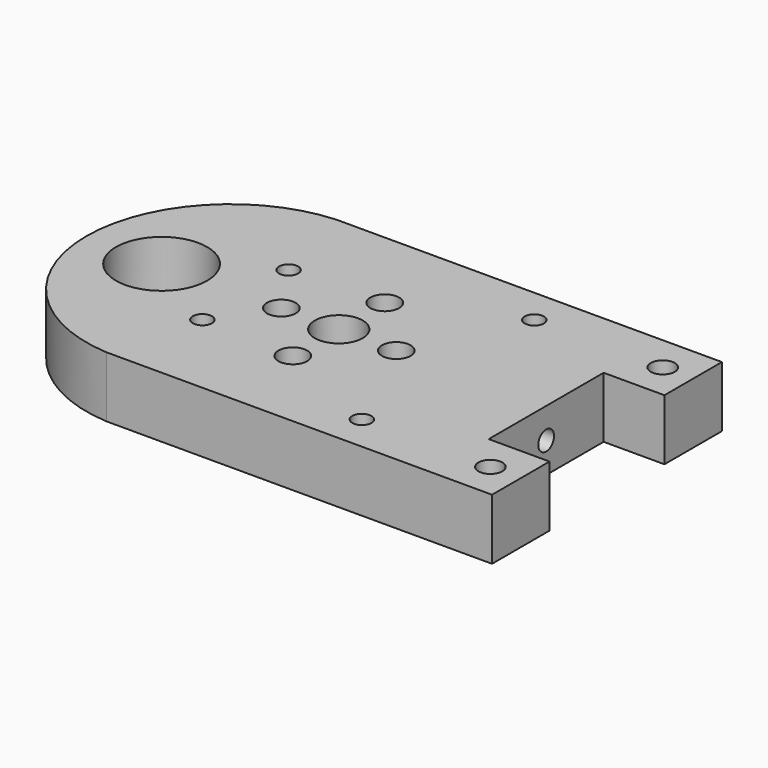
from build123d import *

# Parameters (mm, degrees)
F0_R           = 1.5
F0_R_2         = 4.7625
F1_DEPTH       = 6.35
F2_D           = 2.5
F2_CSINK_D     = 4.7
F2_CSINK_ANGLE = 90
F4_D           = 2.05
F4_DEPTH       = 12.5
F4_TIP         = 0.6158821345
F5_D           = 2
F5_DEPTH       = 8
F5_TIP         = 0.600860619
F7_D           = 2
F7_DEPTH       = 8
F7_TIP         = 0.600860619


# Not quite as in the source:
# - a length typed as a fraction of an inch, garbled in the dataset ("3 / 203.2 mm" for 3/8 in), is restored


with BuildPart() as f1:
    # F0 (on Top) → F1 (new body)
    with BuildSketch(Plane.XY):
        with BuildLine():
            Line((28, 15), (-12.25, 15))
            ThreePointArc((-12.25, 15), (-26.35, 0), (-12.25, -15))
            Line((-12.25, -15), (28, -15))
            Line((28, -15), (28, -7.5))
            Line((28, -7.5), (21.65, -7.5))
            Line((21.65, -7.5), (21.65, 7.5))
            Line((21.65, 7.5), (28, 7.5))
            Line((28, 7.5), (28, 15))
        make_face()
        with Locations((0, -6)):
            Circle(F0_R, mode=Mode.SUBTRACT)
        with Locations((-18.5013860464, 0)):
            Circle(F0_R_2, mode=Mode.SUBTRACT)
        with BuildLine():
            ThreePointArc((-7.5, 0), (-6, 1.5), (-4.5, 0))
            ThreePointArc((-4.5, 0), (-6, -1.5), (-7.5, 0))
        make_face(mode=Mode.SUBTRACT)
        with BuildLine():
            ThreePointArc((2.5, 0), (0, -2.5), (-2.5, 0))
            ThreePointArc((-2.5, 0), (0, 2.5), (2.5, 0))
        make_face(mode=Mode.SUBTRACT)
        with Locations((0, 6)):
            Circle(F0_R, mode=Mode.SUBTRACT)
        with Locations((6, 0)):
            Circle(F0_R, mode=Mode.SUBTRACT)
    extrude(amount=F1_DEPTH)

    # F2 (through all)
    with Locations(Plane(origin=(0, 0, 0), x_dir=(1, 0, 0), z_dir=(0, 0, -1))):
        with Locations((24.825, -11.25), (24.825, 11.25)):
            CounterSinkHole(F2_D / 2, F2_CSINK_D / 2, counter_sink_angle=F2_CSINK_ANGLE)

    # F4
    with Locations(Plane.YZ.offset(21.65)):
        with Locations((0, 3.175)):
            Hole(F4_D / 2, depth=F4_DEPTH)
            with Locations((0, 0, -(F4_DEPTH + F4_TIP / 2))):  # 118° drill point
                Cone(0, F4_D / 2, F4_TIP, mode=Mode.SUBTRACT)

    # F5
    with Locations(Plane(origin=(0, 0, 0), x_dir=(1, 0, 0), z_dir=(0, 0, -1))):
        with Locations((-9.7427857926, 5.625), (-9.7427857926, -5.625)):
            Hole(F5_D / 2, depth=F5_DEPTH)
            with Locations((0, 0, -(F5_DEPTH + F5_TIP / 2))):  # 118° drill point
                Cone(0, F5_D / 2, F5_TIP, mode=Mode.SUBTRACT)

    # F7
    with Locations(Plane.XY.offset(6.35)):
        with Locations((11.4125, -11.25), (11.4125, 11.25)):
            Hole(F7_D / 2, depth=F7_DEPTH)
            with Locations((0, 0, -(F7_DEPTH + F7_TIP / 2))):  # 118° drill point
                Cone(0, F7_D / 2, F7_TIP, mode=Mode.SUBTRACT)


solid = f1.part
